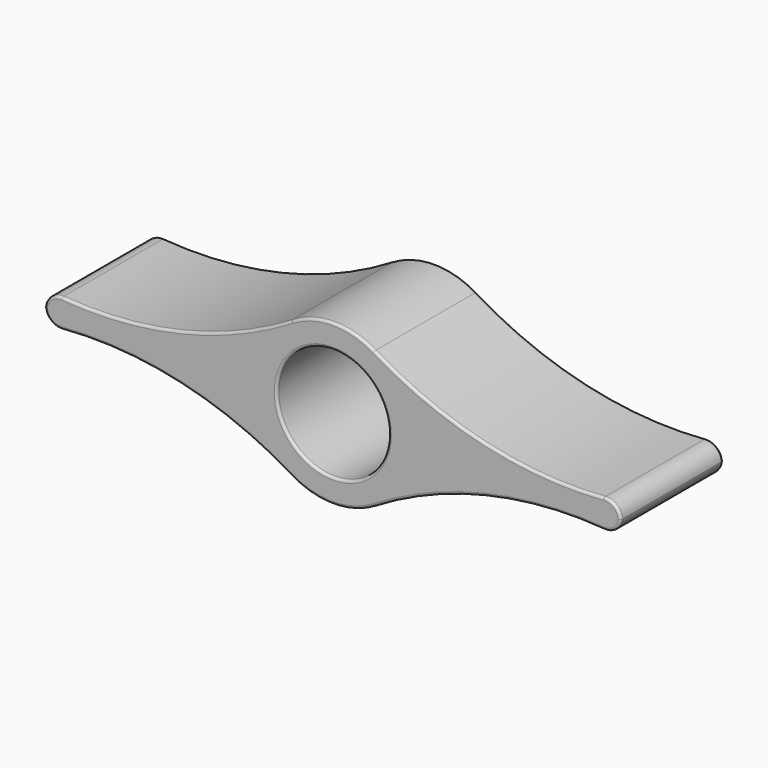
from build123d import *

# Parameters (mm, degrees)
F0_R        = 11.1125
F1_DEPTH    = 25.4
F2_T1_DEPTH = 42.98370548
F3_R        = 0.508


# Not quite as in the source:
# - a fillet or chamfer that OpenCascade refuses, or shapes differently, is made with other operations: its cross-section is extruded or revolved along the edge and cut away or added


with BuildPart() as f1:
    # F0 (on Front) → F1 (new body)
    with BuildSketch(Plane.XZ):
        with BuildLine():
            ThreePointArc((-33.3693444663, 13.6158373531), (-27.7576647521, 19.4023003087), (-25.711236319, 27.1988529712))
            ThreePointArc((-25.711236319, 27.1988529712), (-27.7576647521, 34.9954056337), (-33.3693444663, 40.7818685893))
            ThreePointArc((-33.3693444663, 40.7818685893), (-41.586236319, 43.0738529712), (-49.8031281716, 40.7818685893))
            ThreePointArc((-49.8031281716, 40.7818685893), (-57.461236319, 27.1988529712), (-49.8031281716, 13.6158373531))
            ThreePointArc((-49.8031281716, 13.6158373531), (-41.586236319, 11.3238529712), (-33.3693444663, 13.6158373531))
        make_face()
        with Locations((-41.586236319, 27.1988529712)):
            Circle(F0_R, mode=Mode.SUBTRACT)
        with BuildLine():
            ThreePointArc((-33.3693444663, 40.7818685893), (-27.7576647521, 34.9954056337), (-25.711236319, 27.1988529712))
            ThreePointArc((-25.711236319, 27.1988529712), (-27.7576647521, 19.4023003087), (-33.3693444663, 13.6158373531))
            ThreePointArc((-33.3693444663, 13.6158373531), (-9.7812806597, 22.9500521891), (15.563763681, 24.0238529712))
            Line((15.563763681, 24.0238529712), (15.563763681, 27.1988529712))
            Line((15.563763681, 27.1988529712), (15.563763681, 30.3738529712))
            ThreePointArc((15.563763681, 30.3738529712), (-9.7812806597, 31.4476537533), (-33.3693444663, 40.7818685893))
        make_face()
        with BuildLine():
            ThreePointArc((-49.8031281716, 13.6158373531), (-57.461236319, 27.1988529712), (-49.8031281716, 40.7818685893))
            ThreePointArc((-49.8031281716, 40.7818685893), (-73.3911919783, 31.4476537533), (-98.736236319, 30.3738529712))
            Line((-98.736236319, 30.3738529712), (-98.736236319, 27.1988529712))
            Line((-98.736236319, 27.1988529712), (-98.736236319, 24.0238529712))
            ThreePointArc((-98.736236319, 24.0238529712), (-73.3911919783, 22.9500521891), (-49.8031281716, 13.6158373531))
        make_face()
    extrude(amount=F1_DEPTH)

    # F2: fillet of radius 3.175 on 4 edges, made by hand

    # F2_s2 → F2_t1 (cut)
    with BuildSketch(Plane.XZ.offset(-8.79185274)):
        with BuildLine():
            ThreePointArc((15.563763681, 26.8571118752), (14.5426395524, 29.1898021098), (12.1360825908, 30.0220411424))
            ThreePointArc((12.1360825908, 30.0220411424), (13.8519119629, 30.1785700373), (15.563763681, 30.3738529712))
            Line((15.563763681, 30.3738529712), (15.563763681, 26.8571118752))
        make_face()
        with BuildLine():
            ThreePointArc((12.1360825908, 24.3756648), (14.5426395524, 25.2079038326), (15.563763681, 27.5405940672))
            Line((15.563763681, 27.5405940672), (15.563763681, 24.0238529712))
            ThreePointArc((15.563763681, 24.0238529712), (13.8519119629, 24.219135905), (12.1360825908, 24.3756648))
        make_face()
        with BuildLine():
            ThreePointArc((-95.3085552288, 30.0220411424), (-97.7151121904, 29.1898021098), (-98.736236319, 26.8571118752))
            Line((-98.736236319, 26.8571118752), (-98.736236319, 30.3738529712))
            ThreePointArc((-98.736236319, 30.3738529712), (-97.0243846009, 30.1785700373), (-95.3085552288, 30.0220411424))
        make_face()
        with BuildLine():
            ThreePointArc((-98.736236319, 27.5405940672), (-97.7151121904, 25.2079038326), (-95.3085552288, 24.3756648))
            ThreePointArc((-95.3085552288, 24.3756648), (-97.0243846009, 24.219135905), (-98.736236319, 24.0238529712))
            Line((-98.736236319, 24.0238529712), (-98.736236319, 27.5405940672))
        make_face()
    extrude(amount=F2_T1_DEPTH, mode=Mode.SUBTRACT)

    # F3
    f3_edges = [f1.edges().sort_by_distance(p)[0] for p in [
        (-71.710097, -25.4, 31.825135),
        (-11.462375, 0, 31.825135),
        (-11.462375, -25.4, 22.572571),
        (-11.462375, 0, 22.572571),
        (-52.698736, -25.4, 27.198853),
        (-52.698736, 0, 27.198853),
    ]]
    fillet(f3_edges, radius=F3_R)


solid = f1.part
